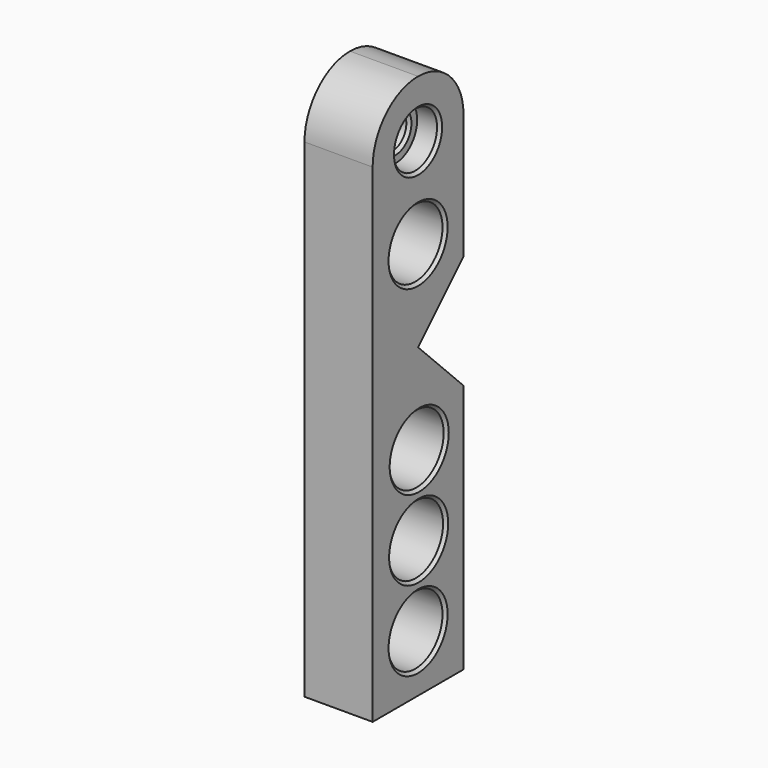
from build123d import *

# Parameters (mm, degrees)
F0_W     = 19.05
F0_H     = 152.4
F1_DEPTH = 31.75
F8_R     = 7.62
F2_DEPTH = 6.35
F3_R     = 4.826
F9_DEPTH = 12.7
F4_R     = 15.87499
F5_DEPTH = 19.05
F8_R_2   = 9.525
F6_DEPTH = 19.05
F7_SIZE  = 0.79375


# Not quite as in the source:
# - a fillet or chamfer is up to 0.001 mm smaller than in the source, because OpenCascade refuses the exact size


with BuildPart() as f1:
    # F0 (on Front) → F1 (new body)
    with BuildSketch(Plane.XZ):
        Rectangle(F0_W, F0_H)
    extrude(amount=F1_DEPTH)

    # F8 (on face) → F2 (cut)
    with BuildSketch(Plane.YZ.offset(9.525)):
        with Locations((-15.875, 60.325)):
            Circle(F8_R)
    extrude(amount=-F2_DEPTH, mode=Mode.SUBTRACT)

    # F3 (on face) → F9 (cut, through all)
    with BuildSketch(Plane.YZ.offset(3.175)):
        with Locations((-15.875, 60.325)):
            Circle(F3_R)
    extrude(amount=-F9_DEPTH, mode=Mode.SUBTRACT)

    # F4 (radius 15.875 in the source; OpenCascade refuses exactly that, so slightly less here)
    f4_edges = [f1.edges().sort_by_distance(p)[0] for p in [
        (0, -31.75, 76.2),
        (0, 0, 76.2),
    ]]
    fillet(f4_edges, radius=F4_R)

    # F8 (on face) → F5 (cut, through all)
    with BuildSketch(Plane.YZ.offset(9.525)):
        Polygon((0, 25.4), (-15.875, 9.525), (0, -6.35), align=None)
    extrude(amount=-F5_DEPTH, mode=Mode.SUBTRACT)

    # F8 (on face) → F6 (cut, through all)
    with BuildSketch(Plane.YZ.offset(9.525)):
        with Locations((-15.875, 34.925)):
            Circle(F8_R_2)
        with Locations((-15.4730585432, -15.8768173255)):
            Circle(F8_R_2)
        with Locations((-15.6740292716, -38.1009086628)):
            Circle(F8_R_2)
        with Locations((-15.875, -60.325)):
            Circle(F8_R_2)
    extrude(amount=-F6_DEPTH, mode=Mode.SUBTRACT)

    # F7
    f7_edges = [f1.edges().sort_by_distance(p)[0] for p in [
        (0, -6.35, 34.925),
        (9.525, -25.4, 34.925),
        (-9.525, -25.4, 34.925),
        (0, -5.948059, -15.876817),
        (9.525, -24.998059, -15.876817),
        (-9.525, -24.998059, -15.876817),
        (0, -6.149029, -38.100909),
        (9.525, -25.199029, -38.100909),
        (-9.525, -25.199029, -38.100909),
        (0, -6.35, -60.325),
        (9.525, -25.4, -60.325),
        (-9.525, -25.4, -60.325),
        (9.525, -23.495, 60.325),
        (-3.175, -11.049, 60.325),
        (3.175, -20.701, 60.325),
        (-9.525, -20.701, 60.325),
    ]]
    chamfer(f7_edges, length=F7_SIZE)


solid = f1.part
